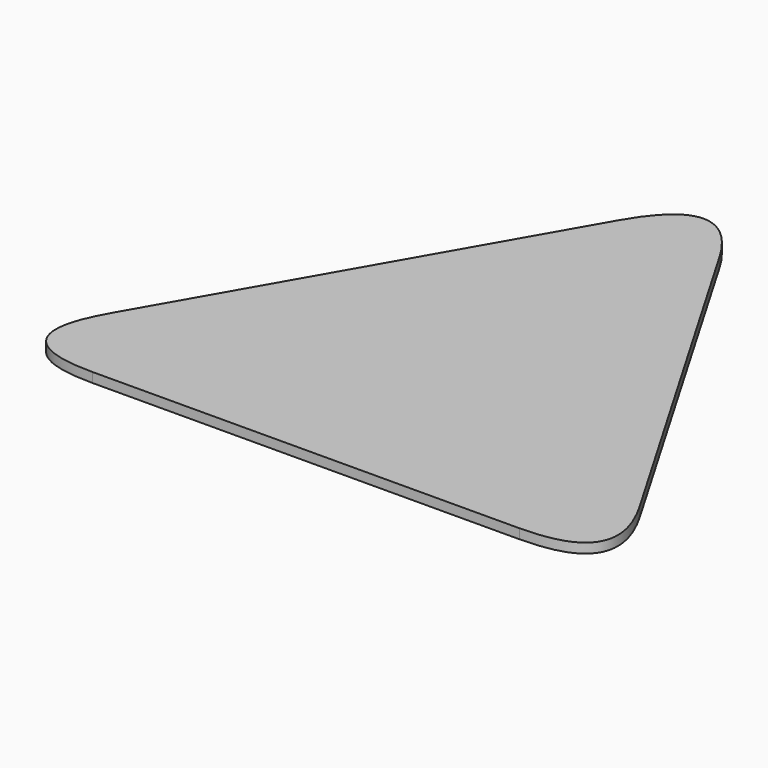
from build123d import *

# Parameters (mm, degrees)
F1_DEPTH    = 5
F2_T1_DEPTH = 264.8076211353


# Not quite as in the source:
# - a fillet or chamfer that OpenCascade refuses, or shapes differently, is made with other operations: its cross-section is extruded or revolved along the edge and cut away or added


with BuildPart() as f1:
    # F0 (on Top) → F1 (new body)
    with BuildSketch(Plane.XY):
        Polygon((-0.6416016338, 191.2437425446), (-161.12652421, -89.6207541227), (162.3517262131, -88.1725256644), align=None)
    extrude(amount=F1_DEPTH)

    # F2: fillet of radius 30 on 3 edges, made by hand

    # F2_s2 → F2_t1 (cut)
    with BuildSketch(Plane.XY.offset(-129.9038105677)):
        with BuildLine():
            add(Edge.make_bspline(
                [(25.5403653575, 146.3605095453), (-0.6416016338, 191.2437425446), (-26.4206381195, 146.1278775095)],
                knots=[0, 0, 0, 1, 1, 1], degree=2, weights=[1, 1, 1]))
            Line((-26.4206381195, 146.1278775095), (-0.6416016338, 191.2437425446))
            Line((-0.6416016338, 191.2437425446), (25.5403653575, 146.3605095453))
        make_face()
        with BuildLine():
            add(Edge.make_bspline(
                [(-135.3474877243, -44.5048890876), (-161.12652421, -89.6207541227), (-109.165520733, -89.3881220869)],
                knots=[0, 0, 0, 1, 1, 1], degree=2, weights=[1, 1, 1]))
            Line((-109.165520733, -89.3881220869), (-161.12652421, -89.6207541227))
            Line((-161.12652421, -89.6207541227), (-135.3474877243, -44.5048890876))
        make_face()
        with BuildLine():
            add(Edge.make_bspline(
                [(136.1697592218, -43.2892926651), (162.3517262131, -88.1725256644), (110.3907227362, -88.4051577003)],
                knots=[0, 0, 0, 1, 1, 1], degree=2, weights=[1, 1, 1]))
            Line((110.3907227362, -88.4051577003), (162.3517262131, -88.1725256644))
            Line((162.3517262131, -88.1725256644), (136.1697592218, -43.2892926651))
        make_face()
    extrude(amount=F2_T1_DEPTH, mode=Mode.SUBTRACT)


solid = f1.part
